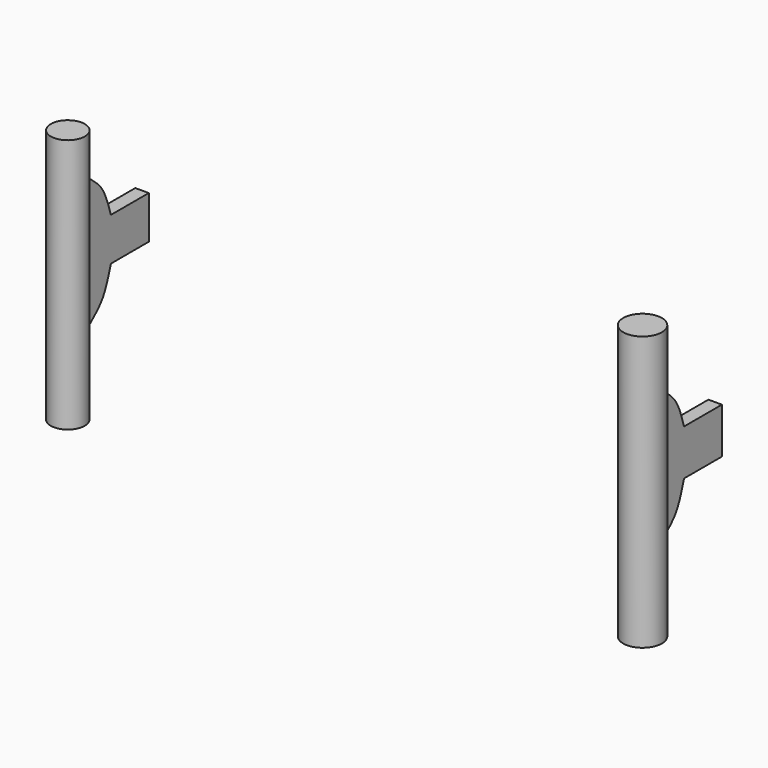
from build123d import *

# Parameters (mm, degrees)
F15_R     = 2.2335856761
F16_DEPTH = 33.528
F17_R     = 2.5454196351
F18_DEPTH = 36.068
F21_DEPTH = 1.778
F24_DEPTH = 1.778


# Not quite as in the source:
# - the program builds the solid bodies; features that only make, move or delete a surface that nothing else refers to are left out


with BuildPart() as f16:
    # F15 (on offset) → F16 (new body)
    with BuildSketch(Plane.XY.offset(34.036)):
        with Locations((-32.7947326005, -12.3348757625)):
            Circle(F15_R)
    extrude(amount=-F16_DEPTH)


with BuildPart() as f18:
    # F17 (on Top) → F18 (new body)
    with BuildSketch(Plane.XY):
        with Locations((42.8683161736, -12.3544856906)):
            Circle(F17_R)
    extrude(amount=F18_DEPTH)

    # F23 (on offset) → F24 (join)
    with BuildSketch(Plane.YZ.offset(41.656)):
        with BuildLine():
            add(Edge.make_bspline(
                [(-9.8325097933, 27.6496764272), (-9.0307658036, 27.0274098331), (-7.333639855, 25.7102003531), (-6.6161287383, 23.2921278525), (-6.237579044, 22.0163837075)],
                knots=[0, 0, 0, 0, 0.4724127814, 1, 1, 1, 1], degree=3))
            Line((-9.8325097933, 27.6496764272), (-9.7397938371, 19.0057530999))
            Line((-9.7397938371, 19.0057530999), (-9.8325097933, 10.3618297726))
            add(Edge.make_bspline(
                [(-9.8325097933, 10.3618297726), (-9.0307658036, 10.9840963667), (-7.333639855, 12.3013058467), (-6.6161287383, 14.7193783474), (-6.237579044, 15.9951224923)],
                knots=[0, 0, 0, 0, 0.4724127814, 1, 1, 1, 1], degree=3))
            Line((-6.237579044, 15.9951224923), (0, 15.9951224923))
            Line((0, 15.9951224923), (0, 19.0057530999))
            Line((0, 19.0057530999), (0, 22.0163837075))
            Line((0, 22.0163837075), (-6.237579044, 22.0163837075))
        make_face()
    extrude(amount=F24_DEPTH)


with BuildPart() as f21:
    # F20 (on offset) → F21 (new body)
    with BuildSketch(Plane.YZ.offset(-33.782)):
        with BuildLine():
            add(Edge.make_bspline(
                [(-9.7659286112, 27.6505146176), (-8.9921918233, 27.024105619), (-7.3467405515, 25.6919659306), (-6.6207069657, 23.2803554227), (-6.2360744923, 22.0027510077)],
                knots=[0, 0, 0, 0, 0.4702277126, 1, 1, 1, 1], degree=3))
            Line((-9.7659286112, 27.6505146176), (-9.7659286112, 10.7072200626))
            add(Edge.make_bspline(
                [(-9.7659286112, 10.7072200626), (-8.9921918233, 11.3336290612), (-7.3467405515, 12.6657687496), (-6.6207069657, 15.0773792575), (-6.2360744923, 16.3549836725)],
                knots=[0, 0, 0, 0, 0.4702277126, 1, 1, 1, 1], degree=3))
            Line((-6.2360744923, 16.3549836725), (0, 16.3549836725))
            Line((0, 16.3549836725), (0, 19.1788673401))
            Line((0, 19.1788673401), (0, 22.0027510077))
            Line((0, 22.0027510077), (-6.2360744923, 22.0027510077))
        make_face()
    extrude(amount=F21_DEPTH)


solid = Compound([f16.part, f18.part, f21.part])
